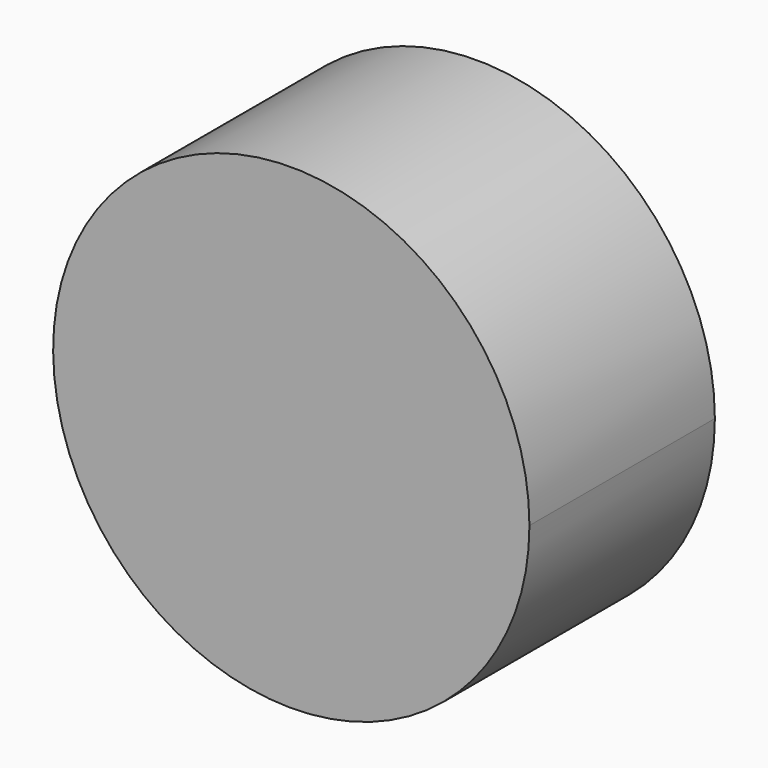
from build123d import *

# Parameters (mm, degrees)
F1_DEPTH = 146


with BuildPart() as f1:
    # F0 (on Front) → F1 (new body)
    with BuildSketch(Plane.XZ):
        with BuildLine():
            ThreePointArc((98.5713273934, -136.5633044432), (205.4788119459, -93.094750199), (249.8745634841, 13.4310340356))
            ThreePointArc((249.8745634841, 13.4310340356), (40.2323620084, 151.0639073005), (-2.6962072245, -96.0186667235))
            ThreePointArc((-2.6962072245, -96.0186667235), (44.121364167, -125.8226221674), (98.5713273934, -136.5633044432))
        make_face()
    extrude(amount=F1_DEPTH)


solid = f1.part
